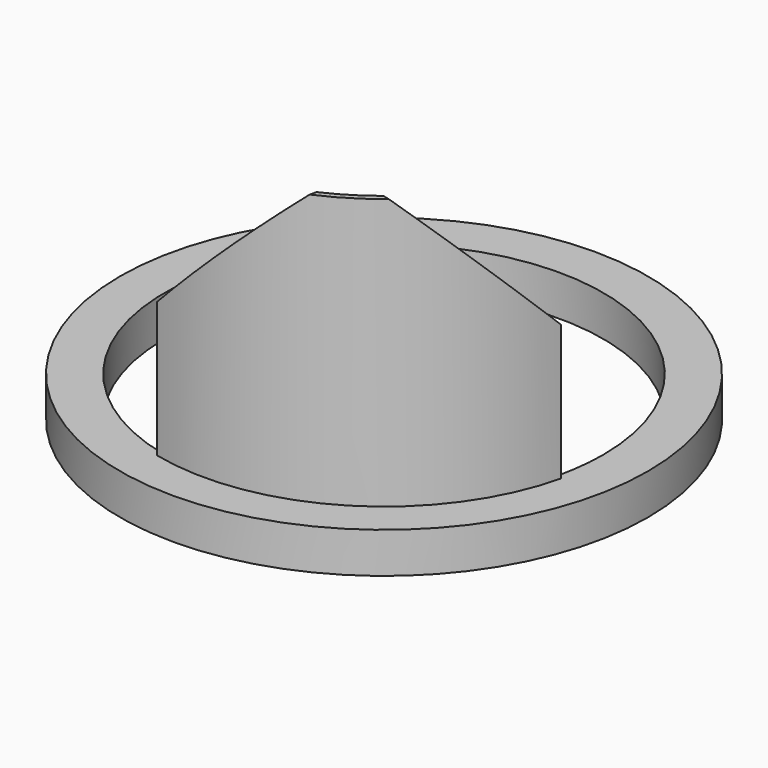
from build123d import *

# Parameters (mm, degrees)
F1_DEPTH    = 20
F2_R        = 19.5
F2_R_2      = 16.2
F3_DEPTH    = 3
F4_T1_DEPTH = 51.8336597593
F4_T3_DEPTH = 51.8336597593


# Not quite as in the source:
# - a fillet or chamfer that OpenCascade refuses, or shapes differently, is made with other operations: its cross-section is extruded or revolved along the edge and cut away or added


with BuildPart() as f1:
    # F0 (on Top) → F1 (new body)
    with BuildSketch(Plane.XY):
        with BuildLine():
            ThreePointArc((15.7618937877, -3.7420187366), (8.4993351577, -13.7913488056), (-3.7420187366, -15.7618937877))
            Line((-3.7420187366, -15.7618937877), (-3.8344142609, -16.1510763504))
            ThreePointArc((-3.8344142609, -16.1510763504), (8.709195285, -14.1318759366), (16.1510763504, -3.8344142609))
            Line((16.1510763504, -3.8344142609), (15.7618937877, -3.7420187366))
        make_face()
    extrude(amount=F1_DEPTH)

    # F2 (on Top) → F3 (join)
    with BuildSketch(Plane.XY):
        Circle(F2_R)
        Circle(F2_R_2, mode=Mode.SUBTRACT)
    extrude(amount=-F3_DEPTH)

    # F4: chamfer of 10 on 2 edges, made by hand

    # F4_s2 → F4_t1 (cut)
    with BuildSketch(Plane(origin=(41.1724307405, -9.7747142149, 0), x_dir=(0, 0, 1), z_dir=(-0.9729564066, 0.2309888109, 0))):
        Polygon((10, 0), (20, -10), (20, 0), align=None)
    extrude(amount=F4_T1_DEPTH, mode=Mode.SUBTRACT)

    # F4_s4 → F4_t3 (cut)
    with BuildSketch(Plane(origin=(2.1982812174, 9.2594606024, 0), x_dir=(0, 0, 1), z_dir=(-0.2309888109, -0.9729564066, 0))):
        Polygon((10, 0), (20, -10), (20, 0), align=None)
    extrude(amount=F4_T3_DEPTH, mode=Mode.SUBTRACT)


solid = f1.part
